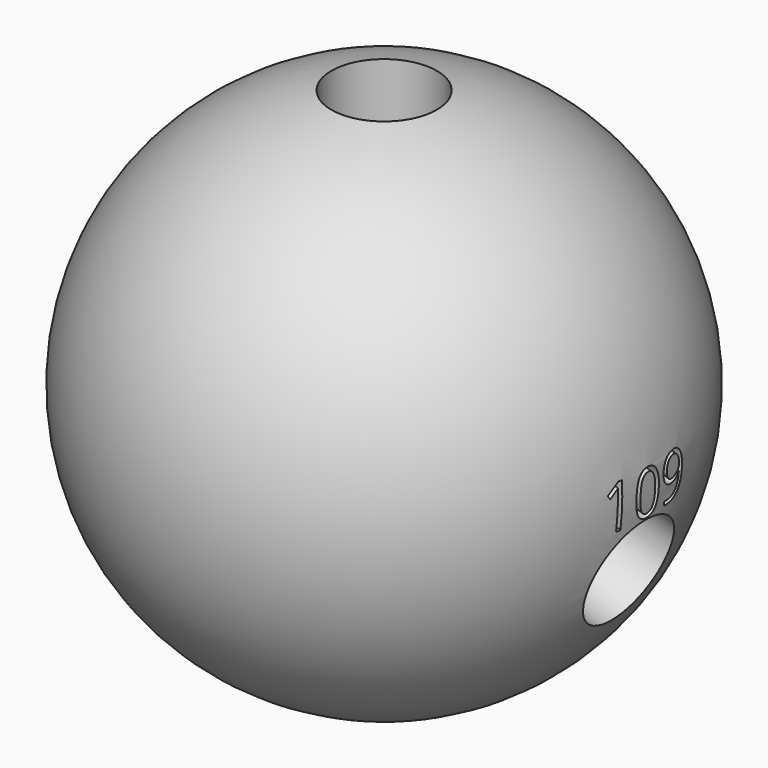
from build123d import *

# Parameters (mm, degrees)
F4_R         = 3.175
F5_DEPTH     = 50.8
F7_ANGLE     = -109
F9_TEXT_SIZE = 3.5851595587
F10_DEPTH    = 19.05


# Not quite as in the source:
# - Text() gives the source's letters only with a copy of the font that has no kerning and outlines rounded to 1/6400 em; it was checked with that copy


with BuildPart() as f2:
    # F0 (on Front) → F2 (revolve)
    with BuildSketch(Plane.XZ):
        with BuildLine():
            Line((0, -15.875), (0, 15.875))
            ThreePointArc((0, 15.875), (-15.875, 0), (0, -15.875))
        make_face()
    revolve(axis=Axis((0, 0, 0), (0, 0, 1)))

    # F9 (on offset) → F10 (cut)
    with BuildSketch(Plane(origin=(24.0161718202, 0, -8.2694311232), x_dir=(0, 1, 0), z_dir=(0.9455185756, 0, -0.3255681545))):
        with Locations((-3.0551978853, 3.2931037713)):
            Text('109', F9_TEXT_SIZE, font='Open Sans', text_align=(TextAlign.LEFT, TextAlign.BOTTOM))
    extrude(amount=-F10_DEPTH, mode=Mode.SUBTRACT)


with BuildPart() as f5:
    # F4 (on offset) → F5 (new body)
    with BuildSketch(Plane.XY.offset(6.35)):
        Circle(F4_R)
    extrude(amount=F5_DEPTH)


with BuildPart() as f7_1:
    # F7: copy of F5
    add(f5.part.rotate(Axis((0, -29.1280634701, 0), (0, -1, 0)), F7_ANGLE))


with BuildPart() as f2_1:
    add(f2.part)

    # F11: cut F5, F7_1
    add(f5.part, mode=Mode.SUBTRACT)
    add(f7_1.part, mode=Mode.SUBTRACT)


solid = f2_1.part
